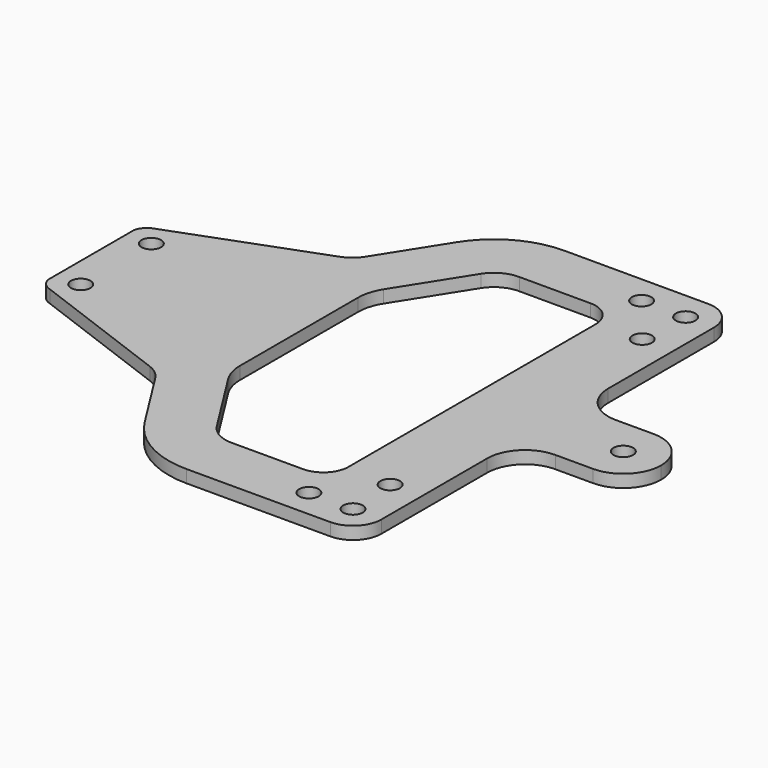
from build123d import *

# Parameters (mm, degrees)
F0_R     = 1.55
F1_DEPTH = 2


# Not quite as in the source:
# - ends of sketch curves that miss each other by under 0.0002 mm in the source are joined


with BuildPart() as f1:
    # F0 (on Top) → F1 (new body)
    with BuildSketch(Plane.XY):
        with BuildLine():
            Line((24.1317584196, 12.0030992724), (24.1317584196, 33.0030992724))
            ThreePointArc((24.1317584196, 33.0030992724), (22.8094861976, 36.1735119864), (19.6355297082, 37.4872550396))
            Line((19.6355297082, 37.4872550396), (-3.1620066842, 37.5062195601))
            ThreePointArc((-3.1620066842, 37.5062195601), (-9.952633868, 35.7733094648), (-15.054516581, 30.9684798394))
            Line((-15.054516581, 30.9684798394), (-21.4377415602, 20.8777601542))
            ThreePointArc((-21.4377415602, 20.8777601542), (-22.515185711, 19.6558592058), (-23.9282391339, 18.8451756363))
            Line((-23.9282391339, 18.8451756363), (-46.5253097099, 10.4110515716))
            ThreePointArc((-46.5253097099, 10.4110515716), (-47.6965598622, 9.7014043841), (-48.3182136925, 8.4811697487))
            Line((-48.3182136925, 8.4811697487), (-48.3182136925, -8.4811697487))
            ThreePointArc((-48.3182136925, -8.4811697487), (-47.6965598622, -9.7014043841), (-46.5253097099, -10.4110515716))
            Line((-46.5253097099, -10.4110515716), (-23.9282391339, -18.8451756363))
            ThreePointArc((-23.9282391339, -18.8451756363), (-22.515185711, -19.6558592058), (-21.4377415602, -20.8777601542))
            Line((-21.4377415602, -20.8777601542), (-15.054516581, -30.9684798394))
            ThreePointArc((-15.054516581, -30.9684798394), (-9.952633868, -35.7733094648), (-3.1620066842, -37.5062195601))
            Line((-3.1620066842, -37.5062195601), (19.6355018203, -37.4872550628))
            ThreePointArc((19.6355018203, -37.4872550628), (22.8150621518, -36.1679133678), (24.1317584196, -32.9872566198))
            Line((24.1317584196, -32.9872566198), (24.1317584196, -12.0030992724))
            Line((24.1317584196, -12.0030992724), (24.1317584196, -12))
            ThreePointArc((24.1317584196, -12), (25.8891177325, -7.7573593129), (30.1317584196, -6))
            Line((30.1317584196, -6), (36.1317584196, -6))
            ThreePointArc((36.1317584196, -6), (40.3733032071, -4.2437363038), (42.1317576192, -0.003099272))
            Line((42.1317576192, -0.003099272), (42.1317584196, 0))
            ThreePointArc((42.1317584196, 0), (40.3743991067, 4.2426406871), (36.1317584196, 6))
            Line((36.1317584196, 6), (30.1317584196, 6))
            ThreePointArc((30.1317584196, 6), (25.8891177325, 7.7573593129), (24.1317584196, 12))
            Line((24.1317584196, 12), (24.1317584196, 12.0030992724))
        make_face()
        with Locations((-44.3682136925, -7)):
            Circle(F0_R, mode=Mode.SUBTRACT)
        with Locations((12.6317863075, -32.9930796663)):
            Circle(F0_R, mode=Mode.SUBTRACT)
        with Locations((19.1317584196, -25)):
            Circle(F0_R, mode=Mode.SUBTRACT)
        with Locations((19.6317863075, -32.9872565966)):
            Circle(F0_R, mode=Mode.SUBTRACT)
        with Locations((-44.3682136925, 7)):
            Circle(F0_R, mode=Mode.SUBTRACT)
        with BuildLine():
            Line((-14.2339508783, 15.4306240067), (-7.4342503505, 26.1797159146))
            ThreePointArc((-7.4342503505, 26.1797159146), (-5.5889861734, 27.9038009834), (-3.1365199939, 28.5061952445))
            Line((-3.1365199939, 28.5061952445), (8.1350859734, 28.4968187664))
            ThreePointArc((8.1350859734, 28.4968187664), (10.9616557954, 27.323776346), (12.1317584196, 24.4959882833))
            Line((12.1317584196, 24.4959882833), (12.1317584196, -24.4985477622))
            ThreePointArc((12.1317584196, -24.4985477622), (10.9611450551, -27.3260150506), (8.1344727862, -28.4985468413))
            Line((8.1344727862, -28.4985468413), (-3.1365199939, -28.5061952445))
            ThreePointArc((-3.1365199939, -28.5061952445), (-5.5889861734, -27.9038009834), (-7.4342503505, -26.1797159146))
            Line((-7.4342503505, -26.1797159146), (-14.2339508783, -15.4306240067))
            ThreePointArc((-14.2339508783, -15.4306240067), (-15.0416860208, -13.6364803831), (-15.3182136925, -11.688424981))
            Line((-15.3182136925, -11.688424981), (-15.3182136925, 11.688424981))
            ThreePointArc((-15.3182136925, 11.688424981), (-15.0416860208, 13.6364803831), (-14.2339508783, 15.4306240067))
        make_face(mode=Mode.SUBTRACT)
        with Locations((36.1317584196, 0)):
            Circle(F0_R, mode=Mode.SUBTRACT)
        with Locations((19.1317584196, 25)):
            Circle(F0_R, mode=Mode.SUBTRACT)
        with Locations((12.6317863075, 32.9930796663)):
            Circle(F0_R, mode=Mode.SUBTRACT)
        with Locations((19.6317863075, 32.9872565966)):
            Circle(F0_R, mode=Mode.SUBTRACT)
    extrude(amount=F1_DEPTH)


solid = f1.part
